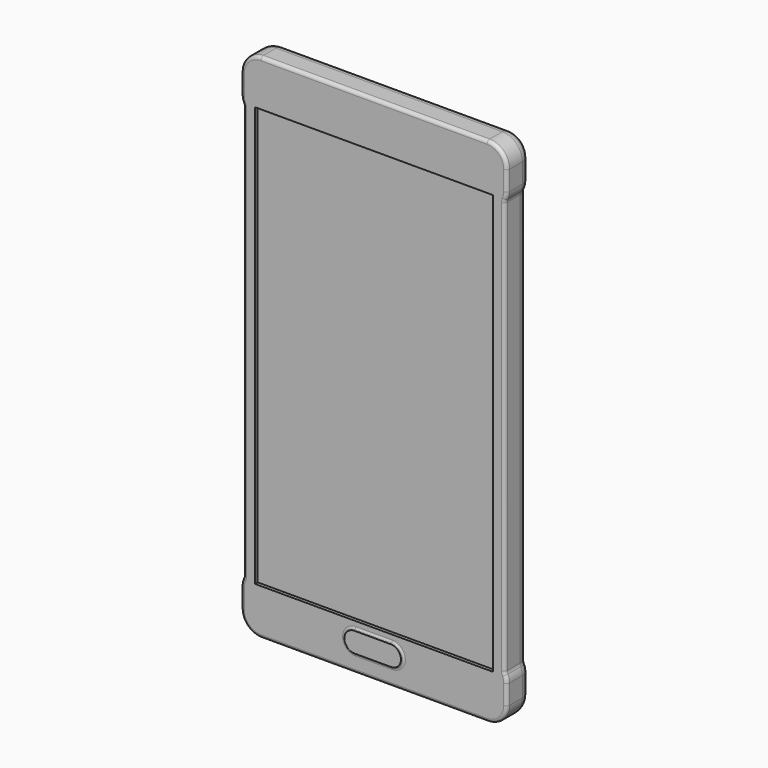
from build123d import *

# Parameters (mm, degrees)
F1_DEPTH     = 9
F3_DEPTH     = 0.5
F4_SIZE      = 0.25
F6_R         = 3.3
F7_T1_DEPTH  = 11
F7_T4_ANGLE  = 180
F7_T6_ANGLE  = 180
F7_T7_DEPTH  = 5.9027099409
F7_T9_DEPTH  = 123.7921215972
F7_T11_DEPTH = 67.9
F7_T13_DEPTH = 5.9027099409
F7_T16_ANGLE = 25.8419327631
F7_T18_ANGLE = 25.8419327632
F7_T20_ANGLE = 90
F7_T22_ANGLE = 25.8419327632
F7_T24_ANGLE = 25.8419327631
F7_T26_ANGLE = 90
F7_T28_ANGLE = 90
F7_T30_ANGLE = 25.8419327631
F7_T32_ANGLE = 25.8419327632
F7_T34_ANGLE = 90
F7_T36_ANGLE = 25.8419327632
F7_T38_ANGLE = 25.8419327631
F9_DEPTH     = 25
F10_R        = 2
F11_W        = 35.75
F11_H        = 63
F12_DEPTH    = 1
F14_DEPTH    = 4


# Not quite as in the source:
# - a fillet or chamfer that OpenCascade refuses, or shapes differently, is made with other operations: its cross-section is extruded or revolved along the edge and cut away or added


with BuildPart() as f1:
    # F0 (on Front) → F1 (new body)
    with BuildSketch(Plane.XZ):
        with BuildLine():
            Line((33.95, 76.85), (33.25, 76.85))
            Line((33.25, 76.85), (-33.25, 76.85))
            Line((-33.25, 76.85), (-33.95, 76.85))
            ThreePointArc((-33.95, 76.85), (-38.1926406871, 75.0926406871), (-39.95, 70.85))
            Line((-39.95, 70.85), (-39.95, 64.9472900591))
            ThreePointArc((-39.95, 64.9472900591), (-39.8233971724, 63.8292560703), (-39.45, 62.7678405873))
            ThreePointArc((-39.45, 62.7678405873), (-39.300641131, 62.3432743941), (-39.25, 61.8960607986))
            Line((-39.25, 61.8960607986), (-39.25, -61.8960607986))
            ThreePointArc((-39.25, -61.8960607986), (-39.300641131, -62.3432743941), (-39.45, -62.7678405873))
            ThreePointArc((-39.45, -62.7678405873), (-39.8233971724, -63.8292560703), (-39.95, -64.9472900591))
            Line((-39.95, -64.9472900591), (-39.95, -70.85))
            ThreePointArc((-39.95, -70.85), (-38.1926406871, -75.0926406871), (-33.95, -76.85))
            Line((-33.95, -76.85), (33.95, -76.85))
            ThreePointArc((33.95, -76.85), (38.1926406871, -75.0926406871), (39.95, -70.85))
            Line((39.95, -70.85), (39.95, -64.9472900591))
            ThreePointArc((39.95, -64.9472900591), (39.8233971724, -63.8292560703), (39.45, -62.7678405873))
            ThreePointArc((39.45, -62.7678405873), (39.300641131, -62.3432743941), (39.25, -61.8960607986))
            Line((39.25, -61.8960607986), (39.25, 61.8960607986))
            ThreePointArc((39.25, 61.8960607986), (39.300641131, 62.3432743941), (39.45, 62.7678405873))
            ThreePointArc((39.45, 62.7678405873), (39.8233971724, 63.8292560703), (39.95, 64.9472900591))
            Line((39.95, 64.9472900591), (39.95, 70.85))
            ThreePointArc((39.95, 70.85), (38.1926406871, 75.0926406871), (33.95, 76.85))
        make_face()
    extrude(amount=F1_DEPTH)

    # F2 (on face) → F3 (join)
    with BuildSketch(Plane.XZ.offset(9)):
        with BuildLine():
            ThreePointArc((8.75, -68.35), (7.7980970389, -66.0519029611), (5.5, -65.1))
            Line((5.5, -65.1), (-5.5, -65.1))
            ThreePointArc((-5.5, -65.1), (-7.7980970389, -66.0519029611), (-8.75, -68.35))
            ThreePointArc((-8.75, -68.35), (-7.7980970389, -70.6480970389), (-5.5, -71.6))
            Line((-5.5, -71.6), (5.5, -71.6))
            ThreePointArc((5.5, -71.6), (7.7980970389, -70.6480970389), (8.75, -68.35))
        make_face()
    extrude(amount=F3_DEPTH)

    # F4
    f4_edges = [f1.edges().sort_by_distance(p)[0] for p in [
        (0, -9.5, -65.1),
        (8.75, -9.5, -68.35),
        (0, -9.5, -71.6),
        (-8.75, -9.5, -68.35),
    ]]
    chamfer(f4_edges, length=F4_SIZE)

    # F6
    f6_edges = [f1.edges().sort_by_distance(p)[0] for p in [
        (0, 0, -76.85),
        (39.823397, 0, 63.829256),
        (39.300641, 0, 62.343274),
        (39.95, 0, 67.898645),
        (39.25, 0, 0),
        (38.192641, 0, 75.092641),
        (39.300641, 0, -62.343274),
        (0, 0, 76.85),
        (39.823397, 0, -63.829256),
        (-38.192641, 0, 75.092641),
        (39.95, 0, -67.898645),
        (-39.95, 0, 67.898645),
        (38.192641, 0, -75.092641),
        (-39.823397, 0, 63.829256),
        (-39.300641, 0, 62.343274),
        (-38.192641, 0, -75.092641),
        (-39.25, 0, 0),
        (-39.95, 0, -67.898645),
        (-39.300641, 0, -62.343274),
        (-39.823397, 0, -63.829256),
    ]]
    fillet(f6_edges, radius=F6_R)

    # F7: fillet of radius 1 on 24 edges, made by hand

    # F7_s2 → F7_t1 (join)
    with BuildSketch(Plane.YZ.offset(-5.5)):
        with BuildLine():
            ThreePointArc((-9, -64.4385621722), (-9.0645856533, -64.7921155628), (-9.25, -65.1))
            Line((-9.25, -65.1), (-9, -65.1))
            Line((-9, -65.1), (-9, -64.4385621722))
        make_face()
        with BuildLine():
            ThreePointArc((-9, -72.2614378278), (-9.0645856533, -71.9078844372), (-9.25, -71.6))
            Line((-9.25, -71.6), (-9, -71.6))
            Line((-9, -71.6), (-9, -72.2614378278))
        make_face()
    extrude(amount=F7_T1_DEPTH)

    # F7_s3 → F7_t4 (revolve)
    with BuildSketch(Plane.YZ.offset(5.5)):
        with BuildLine():
            ThreePointArc((-9, -72.2614378278), (-9.0645856533, -71.9078844372), (-9.25, -71.6))
            Line((-9.25, -71.6), (-9, -71.6))
            Line((-9, -71.6), (-9, -72.2614378278))
        make_face()
    revolve(axis=Axis((5.5, -9, -68.35), (0, -1, 0)), revolution_arc=F7_T4_ANGLE)

    # F7_s5 → F7_t6 (revolve)
    with BuildSketch(Plane.YZ.offset(-5.5)):
        with BuildLine():
            ThreePointArc((-9, -64.4385621722), (-9.0645856533, -64.7921155628), (-9.25, -65.1))
            Line((-9.25, -65.1), (-9, -65.1))
            Line((-9, -65.1), (-9, -64.4385621722))
        make_face()
    revolve(axis=Axis((-5.5, -9, -68.35), (0, -1, 0)), revolution_arc=F7_T6_ANGLE)

    # F7_s8 → F7_t7 (cut)
    with BuildSketch(Plane.XY.offset(64.9472900591)):
        with BuildLine():
            ThreePointArc((38.95, -9), (39.6571067812, -8.7071067812), (39.95, -8))
            Line((39.95, -8), (39.95, -9))
            Line((39.95, -9), (38.95, -9))
        make_face()
        with BuildLine():
            ThreePointArc((-38.95, -9), (-39.6571067812, -8.7071067812), (-39.95, -8))
            Line((-39.95, -8), (-39.95, -9))
            Line((-39.95, -9), (-38.95, -9))
        make_face()
    extrude(amount=F7_T7_DEPTH, mode=Mode.SUBTRACT)

    # F7_s10 → F7_t9 (cut)
    with BuildSketch(Plane.XY.offset(-61.8960607986)):
        with BuildLine():
            ThreePointArc((38.25, -9), (38.9571067812, -8.7071067812), (39.25, -8))
            Line((39.25, -8), (39.25, -9))
            Line((39.25, -9), (38.25, -9))
        make_face()
        with BuildLine():
            ThreePointArc((-38.25, -9), (-38.9571067812, -8.7071067812), (-39.25, -8))
            Line((-39.25, -8), (-39.25, -9))
            Line((-39.25, -9), (-38.25, -9))
        make_face()
    extrude(amount=F7_T9_DEPTH, mode=Mode.SUBTRACT)

    # F7_s12 → F7_t11 (cut)
    with BuildSketch(Plane.YZ.offset(-33.95)):
        with BuildLine():
            ThreePointArc((-9, 75.85), (-8.7071067812, 76.5571067812), (-8, 76.85))
            Line((-8, 76.85), (-9, 76.85))
            Line((-9, 76.85), (-9, 75.85))
        make_face()
        with BuildLine():
            ThreePointArc((-9, -75.85), (-8.7071067812, -76.5571067812), (-8, -76.85))
            Line((-8, -76.85), (-9, -76.85))
            Line((-9, -76.85), (-9, -75.85))
        make_face()
    extrude(amount=F7_T11_DEPTH, mode=Mode.SUBTRACT)

    # F7_s14 → F7_t13 (cut)
    with BuildSketch(Plane.XY.offset(-70.85)):
        with BuildLine():
            ThreePointArc((38.95, -9), (39.6571067812, -8.7071067812), (39.95, -8))
            Line((39.95, -8), (39.95, -9))
            Line((39.95, -9), (38.95, -9))
        make_face()
        with BuildLine():
            ThreePointArc((-38.95, -9), (-39.6571067812, -8.7071067812), (-39.95, -8))
            Line((-39.95, -8), (-39.95, -9))
            Line((-39.95, -9), (-38.95, -9))
        make_face()
    extrude(amount=F7_T13_DEPTH, mode=Mode.SUBTRACT)

    # F7_s15 → F7_t16 (revolve, cut)
    with BuildSketch(Plane(origin=(32.1193806622, 0, 66.3182215748), x_dir=(0, 1, 0), z_dir=(-0.4358898944, 0, -0.9))):
        with BuildLine():
            ThreePointArc((-8, 8.1451325976), (-8.7071067812, 7.8522393788), (-9, 7.1451325976))
            Line((-9, 7.1451325976), (-9, 8.1451325976))
            Line((-9, 8.1451325976), (-8, 8.1451325976))
        make_face()
    revolve(axis=Axis((34.95, -9, 64.9472900591), (0, -1, 0)), revolution_arc=F7_T16_ANGLE, mode=Mode.SUBTRACT)

    # F7_s17 → F7_t18 (revolve, cut)
    with BuildSketch(Plane.XY.offset(61.8960607986)):
        with BuildLine():
            ThreePointArc((39.25, -8), (38.9571067812, -8.7071067812), (38.25, -9))
            Line((38.25, -9), (39.25, -9))
            Line((39.25, -9), (39.25, -8))
        make_face()
    revolve(axis=Axis((41.25, -9, 61.8960607986), (0, 1, 0)), revolution_arc=F7_T18_ANGLE, mode=Mode.SUBTRACT)

    # F7_s19 → F7_t20 (revolve, cut)
    with BuildSketch(Plane.XY.offset(70.85)):
        with BuildLine():
            ThreePointArc((38.95, -9), (39.6571067812, -8.7071067812), (39.95, -8))
            Line((39.95, -8), (39.95, -9))
            Line((39.95, -9), (38.95, -9))
        make_face()
    revolve(axis=Axis((33.95, -9, 70.85), (0, -1, 0)), revolution_arc=F7_T20_ANGLE, mode=Mode.SUBTRACT)

    # F7_s21 → F7_t22 (revolve, cut)
    with BuildSketch(Plane(origin=(32.1193806622, 0, -66.3182215747), x_dir=(0, 1, 0), z_dir=(0.4358898944, 0, -0.9))):
        with BuildLine():
            ThreePointArc((-9, 7.1451325976), (-8.7071067812, 7.8522393788), (-8, 8.1451325976))
            Line((-8, 8.1451325976), (-9, 8.1451325976))
            Line((-9, 8.1451325976), (-9, 7.1451325976))
        make_face()
    revolve(axis=Axis((41.25, -9, -61.8960607986), (0, 1, 0)), revolution_arc=F7_T22_ANGLE, mode=Mode.SUBTRACT)

    # F7_s23 → F7_t24 (revolve, cut)
    with BuildSketch(Plane.XY.offset(-64.9472900591)):
        with BuildLine():
            ThreePointArc((38.95, -9), (39.6571067812, -8.7071067812), (39.95, -8))
            Line((39.95, -8), (39.95, -9))
            Line((39.95, -9), (38.95, -9))
        make_face()
    revolve(axis=Axis((34.95, -9, -64.9472900591), (0, -1, 0)), revolution_arc=F7_T24_ANGLE, mode=Mode.SUBTRACT)

    # F7_s25 → F7_t26 (revolve, cut)
    with BuildSketch(Plane.YZ.offset(-33.95)):
        with BuildLine():
            ThreePointArc((-9, 75.85), (-8.7071067812, 76.5571067812), (-8, 76.85))
            Line((-8, 76.85), (-9, 76.85))
            Line((-9, 76.85), (-9, 75.85))
        make_face()
    revolve(axis=Axis((-33.95, -9, 70.85), (0, -1, 0)), revolution_arc=F7_T26_ANGLE, mode=Mode.SUBTRACT)

    # F7_s27 → F7_t28 (revolve, cut)
    with BuildSketch(Plane.YZ.offset(33.95)):
        with BuildLine():
            ThreePointArc((-9, -75.85), (-8.7071067812, -76.5571067812), (-8, -76.85))
            Line((-8, -76.85), (-9, -76.85))
            Line((-9, -76.85), (-9, -75.85))
        make_face()
    revolve(axis=Axis((33.95, -9, -70.85), (0, -1, 0)), revolution_arc=F7_T28_ANGLE, mode=Mode.SUBTRACT)

    # F7_s29 → F7_t30 (revolve, cut)
    with BuildSketch(Plane.XY.offset(64.9472900591)):
        with BuildLine():
            ThreePointArc((-38.95, -9), (-39.6571067812, -8.7071067812), (-39.95, -8))
            Line((-39.95, -8), (-39.95, -9))
            Line((-39.95, -9), (-38.95, -9))
        make_face()
    revolve(axis=Axis((-34.95, -9, 64.9472900591), (0, -1, 0)), revolution_arc=F7_T30_ANGLE, mode=Mode.SUBTRACT)

    # F7_s31 → F7_t32 (revolve, cut)
    with BuildSketch(Plane(origin=(-32.1193806622, 0, 66.3182215747), x_dir=(0, 1, 0), z_dir=(-0.4358898944, 0, 0.9))):
        with BuildLine():
            ThreePointArc((-9, 7.1451325976), (-8.7071067812, 7.8522393788), (-8, 8.1451325976))
            Line((-8, 8.1451325976), (-9, 8.1451325976))
            Line((-9, 8.1451325976), (-9, 7.1451325976))
        make_face()
    revolve(axis=Axis((-41.25, -9, 61.8960607986), (0, 1, 0)), revolution_arc=F7_T32_ANGLE, mode=Mode.SUBTRACT)

    # F7_s33 → F7_t34 (revolve, cut)
    with BuildSketch(Plane.XY.offset(-70.85)):
        with BuildLine():
            ThreePointArc((-38.95, -9), (-39.6571067812, -8.7071067812), (-39.95, -8))
            Line((-39.95, -8), (-39.95, -9))
            Line((-39.95, -9), (-38.95, -9))
        make_face()
    revolve(axis=Axis((-33.95, -9, -70.85), (0, -1, 0)), revolution_arc=F7_T34_ANGLE, mode=Mode.SUBTRACT)

    # F7_s35 → F7_t36 (revolve, cut)
    with BuildSketch(Plane.XY.offset(-61.8960607986)):
        with BuildLine():
            ThreePointArc((-38.25, -9), (-38.9571067812, -8.7071067812), (-39.25, -8))
            Line((-39.25, -8), (-39.25, -9))
            Line((-39.25, -9), (-38.25, -9))
        make_face()
    revolve(axis=Axis((-41.25, -9, -61.8960607986), (0, 1, 0)), revolution_arc=F7_T36_ANGLE, mode=Mode.SUBTRACT)

    # F7_s37 → F7_t38 (revolve, cut)
    with BuildSketch(Plane(origin=(-32.1193806622, 0, -66.3182215748), x_dir=(0, 1, 0), z_dir=(0.4358898944, 0, 0.9))):
        with BuildLine():
            ThreePointArc((-9, 7.1451325976), (-8.7071067812, 7.8522393788), (-8, 8.1451325976))
            Line((-8, 8.1451325976), (-9, 8.1451325976))
            Line((-9, 8.1451325976), (-9, 7.1451325976))
        make_face()
    revolve(axis=Axis((-34.95, -9, -64.9472900591), (0, -1, 0)), revolution_arc=F7_T38_ANGLE, mode=Mode.SUBTRACT)

    # F8 (on face) → F9 (join)
    with BuildSketch(Plane(origin=(0, 0, -76.85), x_dir=(1, 0, 0), z_dir=(0, 0, -1))):
        with BuildLine():
            add(Edge.make_bspline(
                [(0, 0), (-12.75, 0.0901000897), (-22.6333333333, 2.227253591), (-33.95, 3.3408803865)],
                knots=[0, 0, 0, 0, 34.1139851345, 34.1139851345, 34.1139851345, 34.1139851345], degree=3))
            add(Edge.make_bspline(
                [(0, 0), (12.75, 0.0901000897), (22.6333333333, 2.227253591), (33.95, 3.3408803865)],
                knots=[0, 0, 0, 0, 34.1139851345, 34.1139851345, 34.1139851345, 34.1139851345], degree=3))
            Line((33.95, 3.3408803865), (-33.95, 3.3408803865))
        make_face()
    extrude(amount=-F9_DEPTH)

    # F10
    f10_edges = [f1.edges().sort_by_distance(p)[0] for p in [
        (-16.809598, -1.199631, -76.85),
        (16.809598, -1.199631, -76.85),
    ]]
    fillet(f10_edges, radius=F10_R)

    # F11 (on face) → F12 (cut)
    with BuildSketch(Plane.XZ.offset(9)):
        with Locations((-17.875, 31.5)):
            Rectangle(F11_W, F11_H)
        with Locations((-17.875, -31.5)):
            Rectangle(F11_W, F11_H)
        with Locations((17.875, -31.5)):
            Rectangle(F11_W, F11_H)
        with Locations((17.875, 31.5)):
            Rectangle(F11_W, F11_H)
    extrude(amount=-F12_DEPTH, mode=Mode.SUBTRACT)

    # F13 (on face) → F14 (cut)
    with BuildSketch(Plane(origin=(0, 0, -76.85), x_dir=(1, 0, 0), z_dir=(0, 0, -1))):
        with BuildLine():
            ThreePointArc((3.5, 4.3340018644), (3.2071067812, 5.0411086456), (2.5, 5.3340018644))
            Line((2.5, 5.3340018644), (-2.5, 5.3340018644))
            ThreePointArc((-2.5, 5.3340018644), (-3.2071067812, 5.0411086456), (-3.5, 4.3340018644))
            Line((-3.5, 4.3340018644), (-3.5, 3.3840018644))
            ThreePointArc((-3.5, 3.3840018644), (-3.4267766953, 3.2072251691), (-3.25, 3.1340018644))
            Line((-3.25, 3.1340018644), (3.25, 3.1340018644))
            ThreePointArc((3.25, 3.1340018644), (3.4267766953, 3.2072251691), (3.5, 3.3840018644))
            Line((3.5, 3.3840018644), (3.5, 4.3340018644))
        make_face()
    extrude(amount=-F14_DEPTH, mode=Mode.SUBTRACT)


solid = f1.part
